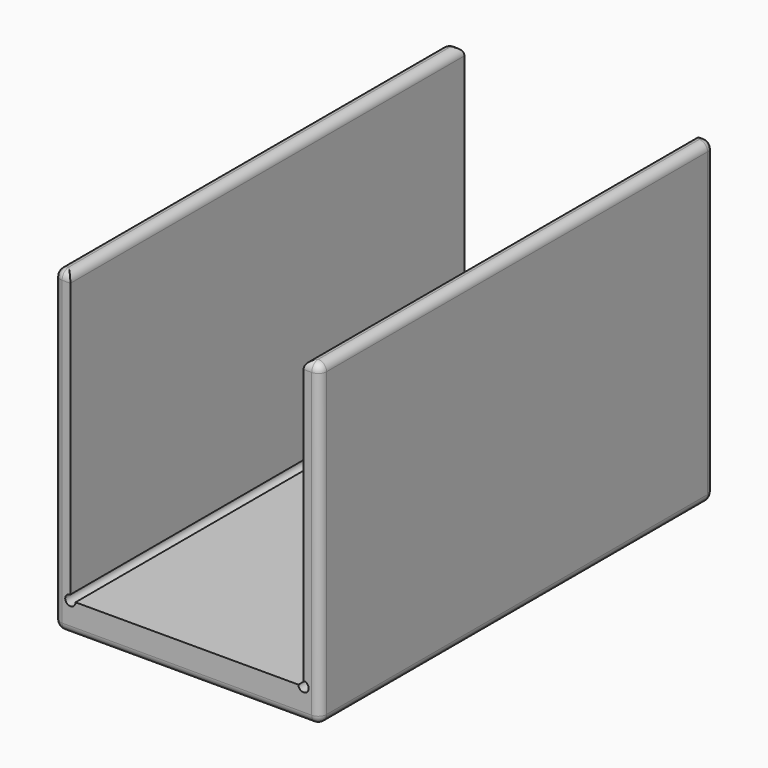
from build123d import *

# Parameters (mm, degrees)
F1_DEPTH = 76.2
F2_R     = 1.26999


# Not quite as in the source:
# - a fillet or chamfer is up to 0.001 mm smaller than in the source, because OpenCascade refuses the exact size


with BuildPart() as f1:
    # F0 (on Front) → F1 (new body)
    with BuildSketch(Plane.XZ):
        with BuildLine():
            Line((-18.034, 19.05), (-20.574, 19.05))
            Line((-20.574, 19.05), (-20.574, -30.1625))
            Line((-20.574, -30.1625), (0, -30.1625))
            Line((0, -30.1625), (0, -25.4))
            Line((0, -25.4), (-17.24025, -25.4))
            ThreePointArc((-17.24025, -25.4), (-18.5952660076, -25.9612660076), (-18.034, -24.60625))
            Line((-18.034, -24.60625), (-18.034, 19.05))
        make_face()
        with BuildLine():
            Line((0, -25.4), (0, -30.1625))
            Line((0, -30.1625), (20.574, -30.1625))
            Line((20.574, -30.1625), (20.574, 19.05))
            Line((20.574, 19.05), (18.034, 19.05))
            Line((18.034, 19.05), (18.034, -24.60625))
            ThreePointArc((18.034, -24.60625), (18.5952660076, -24.8387339924), (18.82775, -25.4))
            ThreePointArc((18.82775, -25.4), (18.034, -26.19375), (17.24025, -25.4))
            Line((17.24025, -25.4), (0, -25.4))
        make_face()
    extrude(amount=F1_DEPTH)

    # F2 (radius 1.27 in the source; OpenCascade refuses exactly that, so slightly less here)
    f2_edges = [f1.edges().sort_by_distance(p)[0] for p in [
        (20.574, -38.1, 19.05),
        (18.034, -38.1, 19.05),
        (19.304, 0, 19.05),
        (19.304, -76.2, 19.05),
        (-18.034, -38.1, 19.05),
        (-20.574, -38.1, 19.05),
        (-19.304, 0, 19.05),
        (-19.304, -76.2, 19.05),
        (-20.574, -76.2, -5.55625),
        (20.574, -76.2, -5.55625),
        (20.574, 0, -5.55625),
        (-20.574, 0, -5.55625),
        (-20.574, -38.1, -30.1625),
        (20.574, -38.1, -30.1625),
        (0, 0, -30.1625),
        (0, -76.2, -30.1625),
    ]]
    fillet(f2_edges, radius=F2_R)


solid = f1.part
